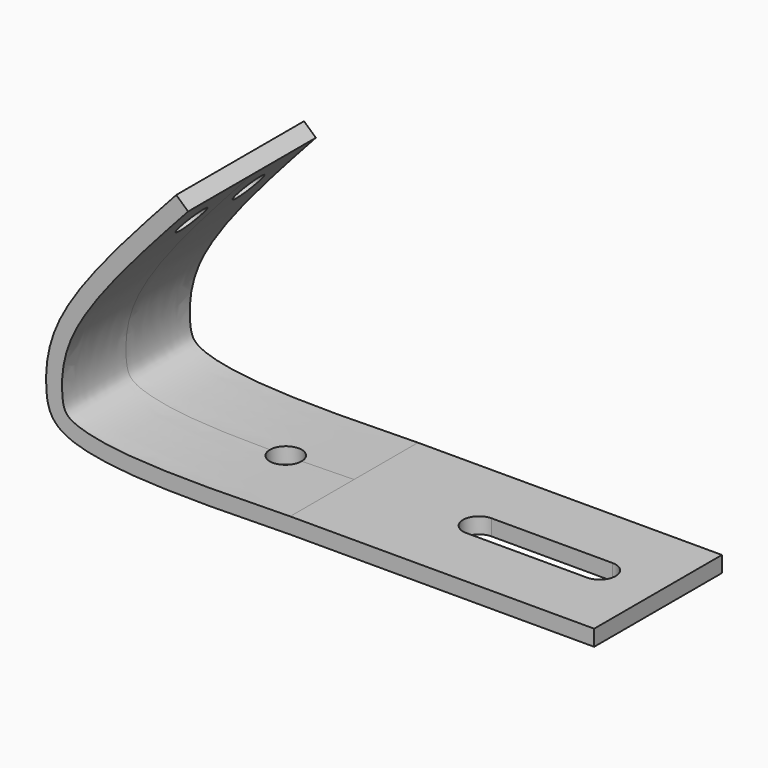
from build123d import *

# Parameters (mm, degrees)
F1_DEPTH = 12.7
F2_R     = 2.5258492874
F3_DEPTH = 25.4
F4_R     = 2.1400235993
F5_DEPTH = 40.4368


# Not quite as in the source:
# - the dataset's text gives a spline's control points without its knots; the knots are read off the source's solid


with BuildPart() as f1:
    # F0 (on Front) → F1 (new body, symmetric)
    with BuildSketch(Plane.XZ):
        with BuildLine():
            Line((0, 0), (48.2959374785, 0))
            Line((48.2959374785, 0), (48.2959374785, 2.5394760895))
            Line((48.2959374785, 2.5394760895), (-0.0515715588, 2.5394760895))
            add(Edge.make_bspline(
                [(-0.0515715588, 2.5394760895), (-2.8119433736, 2.483418591), (-8.3215370793, 2.3715547555), (-14.8862207263, 2.3304431847), (-19.7615353318, 2.4143726599), (-23.1818367267, 2.5495049516), (-26.3158788676, 2.7697262436), (-29.10952047, 3.0860372826), (-31.5014722374, 3.5044696473), (-33.098988631, 3.9348941938), (-34.0920704314, 4.3081791385), (-34.682607858, 4.5911017366), (-35.1013905941, 4.8530355227), (-35.4008518034, 5.1000700078), (-35.6159855159, 5.3347401249), (-35.7819183711, 5.5758159737), (-35.92140655, 5.8508484354), (-36.0425435087, 6.1848616845), (-36.144226957, 6.5923339339), (-36.2237566077, 7.0778496529), (-36.2805057404, 7.637072992), (-36.3193342913, 8.2709875563), (-36.3384695758, 8.9135732532), (-36.3330928413, 9.7914409254), (-36.261643379, 10.9281574681), (-36.0475352681, 12.3685738983), (-35.6775730051, 13.8981724613), (-35.2138687176, 15.2575094864), (-34.7330965193, 16.401242858), (-34.1733102467, 17.5828489424), (-33.3073094378, 19.1595304993), (-31.6019263974, 21.8521800764), (-28.9332176346, 25.4842211074), (-25.0853505789, 30.1375262273), (-20.8028583618, 34.9860832457), (-17.7959736251, 38.2899253259), (-16.2884617416, 39.9462905206)],
                knots=[0, 0, 0, 0, 0.0625, 0.125, 0.15625, 0.1875, 0.21875, 0.25, 0.28125, 0.3125, 0.328125, 0.34375, 0.359375, 0.375, 0.390625, 0.40625, 0.421875, 0.4375, 0.453125, 0.46875, 0.484375, 0.5, 0.515625, 0.53125, 0.5625, 0.59375, 0.625, 0.65625, 0.671875, 0.6875, 0.71875, 0.75, 0.8125, 0.875, 0.9375, 1, 1, 1, 1], degree=3))
            Line((-16.2884617416, 39.9462905206), (-18.1669350713, 41.6559502482))
            add(Edge.make_bspline(
                [(0, 0), (-15.5073129004, -0.3149217675), (-37.2621230556, -0.7567174099), (-39.2536256958, 8.1224977791), (-38.1267092114, 19.7253269875), (-25.887394925, 33.1731640573), (-18.1669350713, 41.6559502482)],
                knots=[0, 0, 0, 0, 0.3511146763, 0.4925697427, 0.679917123, 1, 1, 1, 1], degree=3))
        make_face()
    extrude(amount=F1_DEPTH, both=True)

    # F2 (on face) → F3 (cut)
    with BuildSketch(Plane.XY.offset(2.5394760895)):
        with BuildLine():
            Line((19.808197394, -2.5258492874), (39.0199758112, -2.5258492874))
            ThreePointArc((39.0199758112, -2.5258492874), (41.5458250987, 0), (39.0199758112, 2.5258492874))
            Line((39.0199758112, 2.5258492874), (19.808197394, 2.5258492874))
            ThreePointArc((19.808197394, 2.5258492874), (17.2823481066, 0), (19.808197394, -2.5258492874))
        make_face()
        with Locations((-10.9150968492, 0)):
            Circle(F2_R)
    extrude(amount=-F3_DEPTH, mode=Mode.SUBTRACT)

    # F4 (on Right) → F5 (cut)
    with BuildSketch(Plane.YZ):
        with Locations((6.0327826068, 33.9822471142)):
            Circle(F4_R)
        with Locations((-5.323168356, 33.9822471142)):
            Circle(F4_R)
    extrude(amount=-F5_DEPTH, mode=Mode.SUBTRACT)


solid = f1.part
